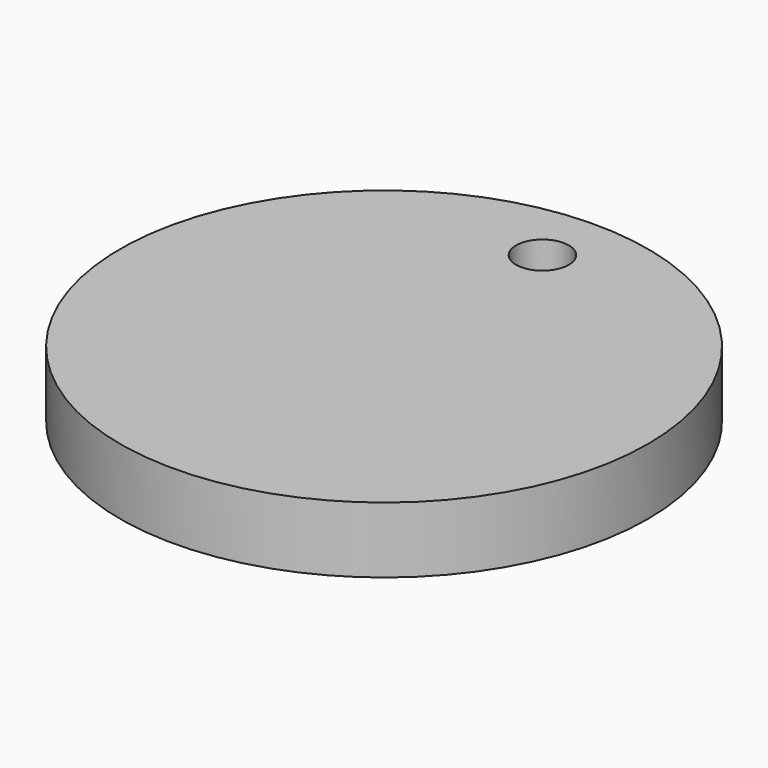
from build123d import *

# Parameters (mm, degrees)
F0_R     = 12.7
F1_DEPTH = 3.175
F2_R     = 1.27
F3_DEPTH = 25.4


# Not quite as in the source:
# - a length typed as a fraction of an inch, garbled in the dataset ("3 / 203.2 mm" for 3/8 in), is restored


with BuildPart() as f1:
    # F0 (on Top) → F1 (new body)
    with BuildSketch(Plane.XY):
        Circle(F0_R)
    extrude(amount=F1_DEPTH)

    # F2 (on face) → F3 (cut)
    with BuildSketch(Plane.XY.offset(3.175)):
        with Locations((0, 9.525)):
            Circle(F2_R)
    extrude(amount=-F3_DEPTH, mode=Mode.SUBTRACT)


solid = f1.part
